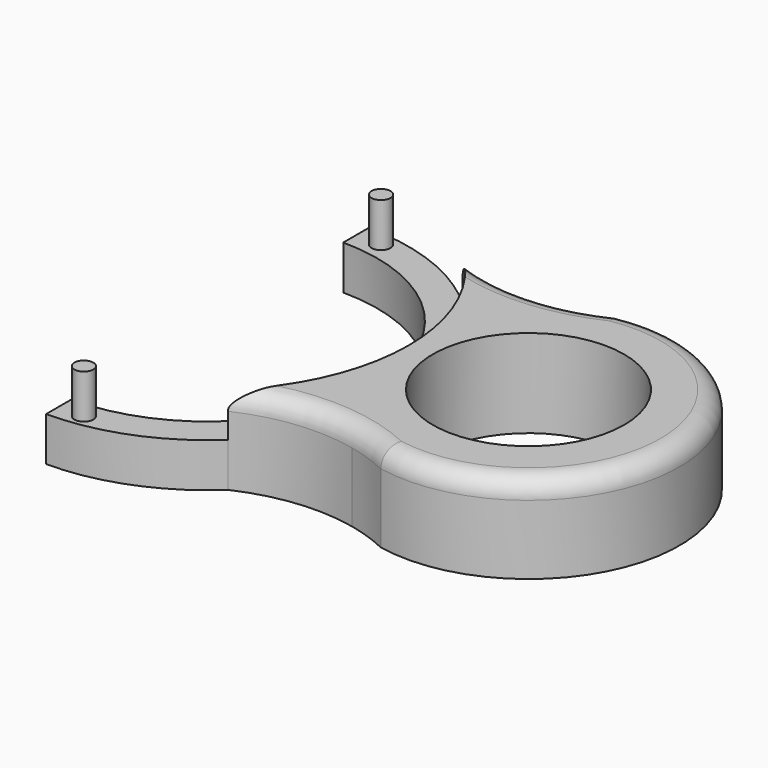
from build123d import *

# Parameters (mm, degrees)
F0_R        = 7.6
F1_DEPTH    = 7
F0_R_2      = 0.75
F2_DEPTH    = 3.5
F3_DEPTH    = 7
F4_T2_ANGLE = 216.4149225178
F4_T4_ANGLE = 62.3523570928
F4_T6_ANGLE = 62.3523570928


# Not quite as in the source:
# - a fillet or chamfer that OpenCascade refuses, or shapes differently, is made with other operations: its cross-section is extruded or revolved along the edge and cut away or added


with BuildPart() as f1:
    # F0 (on Top) → F1 (new body)
    with BuildSketch(Plane.XY):
        with BuildLine():
            ThreePointArc((10.9573513926, 11.6591788072), (14.6853263886, 6.3514713932), (16, 0))
            ThreePointArc((16, 0), (14.6853263886, -6.3514713932), (10.9573513926, -11.6591788072))
            ThreePointArc((10.9573513926, -11.6591788072), (15.4193407408, -10.4308709156), (20.0404607585, -10.6825433249))
            ThreePointArc((20.0404607585, -10.6825433249), (21.6577434142, -11.137707206), (23.2109449826, -11.7782868144))
            ThreePointArc((23.2109449826, -11.7782868144), (37.5070198327, 0), (23.2109449826, 11.7782868144))
            ThreePointArc((23.2109449826, 11.7782868144), (21.6577434142, 11.137707206), (20.0404607585, 10.6825433249))
            ThreePointArc((20.0404607585, 10.6825433249), (15.4193407408, 10.4308709156), (10.9573513926, 11.6591788072))
        make_face()
        with Locations((25.5070198327, 0)):
            Circle(F0_R, mode=Mode.SUBTRACT)
    extrude(amount=F1_DEPTH)

    # F0 (on Top) → F2 (join)
    with BuildSketch(Plane.XY):
        with BuildLine():
            ThreePointArc((10.9573513926, -11.6591788072), (14.6853263886, -6.3514713932), (16, 0))
            ThreePointArc((16, 0), (14.6853263886, 6.3514713932), (10.9573513926, 11.6591788072))
            ThreePointArc((10.9573513926, 11.6591788072), (5.8929253807, 14.875262366), (0, 16))
            Line((0, 16), (0, 13.5))
            ThreePointArc((0, 13.5), (13.5, 0), (0, -13.5))
            Line((0, -13.5), (0, -16))
            ThreePointArc((0, -16), (5.8929253807, -14.875262366), (10.9573513926, -11.6591788072))
        make_face()
        with Locations((2, -14.75)):
            Circle(F0_R_2, mode=Mode.SUBTRACT)
        with Locations((2, 14.75)):
            Circle(F0_R_2, mode=Mode.SUBTRACT)
    extrude(amount=F2_DEPTH)

    # F0 (on Top) → F3 (join)
    with BuildSketch(Plane.XY):
        with Locations((2, -14.75)):
            Circle(F0_R_2)
        with Locations((2, 14.75)):
            Circle(F0_R_2)
    extrude(amount=F3_DEPTH)

    # F4: fillet of radius 1.5 on 3 edges, made by hand

    # F4_s1 → F4_t2 (revolve, cut)
    with BuildSketch(Plane(origin=(23.0167594858, -7.5708469449, 0), x_dir=(0, 0, 1), z_dir=(-0.9499313701, 0.3124586246, 0))):
        with BuildLine():
            ThreePointArc((7, -2.5301116659), (6.5606601718, -3.5907718377), (5.5, -4.0301116659))
            Line((5.5, -4.0301116659), (5.5, -4.0601116659))
            Line((5.5, -4.0601116659), (7.03, -4.0601116659))
            Line((7.03, -4.0601116659), (7.03, -2.5301116659))
            Line((7.03, -2.5301116659), (7, -2.5301116659))
        make_face()
    revolve(axis=Axis((25.5070198327, 0, 7), (0, 0, 1)), revolution_arc=F4_T2_ANGLE, mode=Mode.SUBTRACT)

    # F4_s3 → F4_t4 (revolve, cut)
    with BuildSketch(Plane(origin=(1.7157414838, -1.0154655771, 0), x_dir=(0, 0, 1), z_dir=(-0.8605708042, 0.5093308267, 0))):
        with BuildLine():
            ThreePointArc((7, 14.0363317803), (6.5606601718, 15.0969919521), (5.5, 15.5363317803))
            Line((5.5, 15.5363317803), (5.5, 15.5663317803))
            Line((5.5, 15.5663317803), (7.03, 15.5663317803))
            Line((7.03, 15.5663317803), (7.03, 14.0363317803))
            Line((7.03, 14.0363317803), (7, 14.0363317803))
        make_face()
    revolve(axis=Axis((16.9576039777, 24.7373480679, 7), (0, 0, 1)), revolution_arc=F4_T4_ANGLE, mode=Mode.SUBTRACT)

    # F4_s5 → F4_t6 (revolve, cut)
    with BuildSketch(Plane(origin=(23.3323950061, -14.4290028917, 0), x_dir=(0, 0, 1), z_dir=(0.8505074888, -0.5259629374, 0))):
        with BuildLine():
            ThreePointArc((5.5, -2.2687096081), (6.5606601718, -2.7080494363), (7, -3.7687096081))
            Line((7, -3.7687096081), (7.03, -3.7687096081))
            Line((7.03, -3.7687096081), (7.03, -2.2387096081))
            Line((7.03, -2.2387096081), (5.5, -2.2387096081))
            Line((5.5, -2.2387096081), (5.5, -2.2687096081))
        make_face()
    revolve(axis=Axis((16.9576039777, -24.7373480679, 7), (0, 0, 1)), revolution_arc=F4_T6_ANGLE, mode=Mode.SUBTRACT)


solid = f1.part
